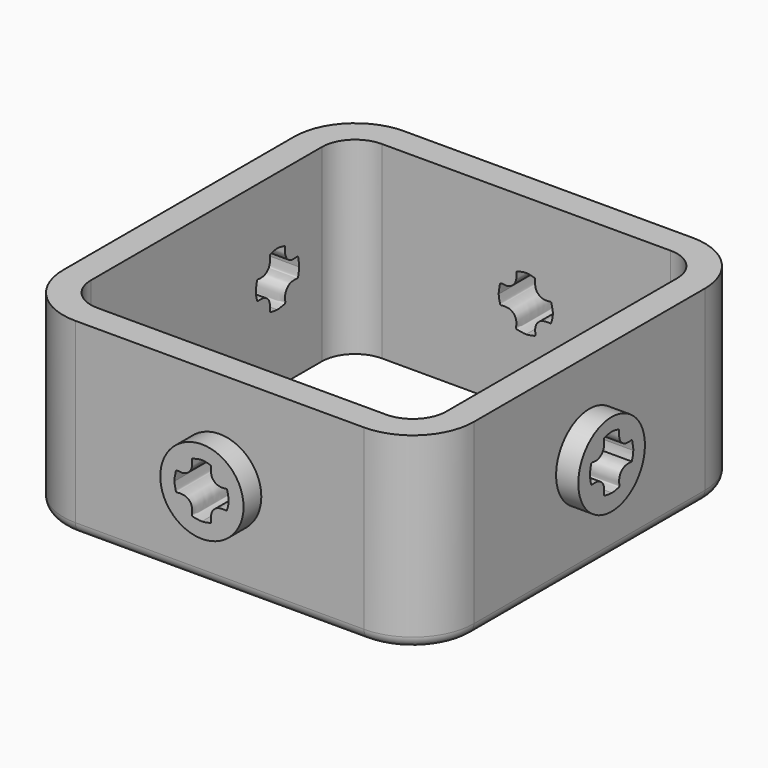
from build123d import *

# Parameters (mm, degrees)
F0_W      = 37
F0_H      = 37
F0_W_2    = 32
F0_H_2    = 32
F1_DEPTH  = 17
F2_R      = 3
F3_R      = 3.75
F4_DEPTH  = 2
F5_R      = 3.75
F6_DEPTH  = 2
F8_DEPTH  = 43.1
F9_R      = 5.5
F10_R     = 1
F12_DEPTH = 19.1
F13_R     = 3.75
F14_DEPTH = 2
F16_DEPTH = 25


# Not quite as in the source:
# - a pattern or mirror of a feature is missing from the dataset's text; its kind, count and spacing are read off the source's solid
# - a feature names something its author has since deleted; it is built from what else it names


with BuildPart() as f1:
    # F0 (on Top) → F1 (new body)
    with BuildSketch(Plane.XY):
        Rectangle(F0_W, F0_H)
        Rectangle(F0_W_2, F0_H_2, mode=Mode.SUBTRACT)
    extrude(amount=F1_DEPTH)

    # F2
    f2_edges = [f1.edges().sort_by_distance(p)[0] for p in [
        (-16, 16, 8.5),
        (16, 16, 8.5),
        (16, -16, 8.5),
        (-16, -16, 8.5),
    ]]
    fillet(f2_edges, radius=F2_R)

    # F3 (on face) → F4 (join)
    with BuildSketch(Plane(origin=(-18.5, 0, 0), x_dir=(0, -1, 0), z_dir=(-1, 0, 0))):
        with Locations((-8, 8.5)):
            Circle(F3_R)
        with BuildLine():
            ThreePointArc((11.75, 8.5), (8, 12.25), (4.25, 8.5))
            ThreePointArc((4.25, 8.5), (8, 4.75), (11.75, 8.5))
        make_face()
    extrude(amount=F4_DEPTH)

    # F5 (on face) → F6 (join)
    with BuildSketch(Plane.XZ.offset(18.5)):
        with Locations((0, 8.5)):
            Circle(F5_R)
    f6 = extrude(amount=F6_DEPTH)

    # F6_copies: F6 across plane
    add(f6.mirror(Plane.ZX))

    # F7 (on face) → F8 (cut)
    with BuildSketch(Plane.XZ.offset(20.5)):
        with BuildLine():
            add(Edge.make_bspline(
                [(-0.8818770875, 10.8338655923), (-0.5842589697, 10.9177265658), (-0.286617976, 11.0030384337), (0.0019111567, 11.0008564852)],
                knots=[0, 0, 0, 0, 0.5095712537, 0.5095712537, 0.5095712537, 0.5095712537], degree=3))
            add(Edge.make_bspline(
                [(-0.8818770875, 10.8338655923), (-0.8820201865, 10.7347613501), (-0.8822944124, 10.5448442864), (-0.8804438019, 10.2880725266), (-0.8966687632, 10.0993117062), (-1.068596367, 9.7410775604), (-1.2714231603, 9.5700618662), (-1.5485520687, 9.4347869785), (-1.8416222457, 9.3826988039), (-2.3755108047, 9.5150016948), (-2.3789289487, 9.1137847523), (-2.4627570935, 8.8526861228), (-2.4717232683, 8.6257526766), (-2.4694705272, 8.5165882094)],
                knots=[0, 0, 0, 0, 0.0273605905, 0.0524320947, 0.0745076412, 0.1056108167, 0.1318649214, 0.158948127, 0.1874687016, 0.220995097, 0.2482860623, 0.2755720453, 0.3045111481, 0.3045111481, 0.3045111481, 0.3045111481], degree=3))
            Line((-2.4694705272, 8.5165882094), (0.0019111567, 8.5165882094))
            Line((0.0019111567, 8.5165882094), (0.0019111567, 11.0008564852))
        make_face()
        with BuildLine():
            add(Edge.make_bspline(
                [(0.0019111567, 11.0008564852), (0.2796014301, 10.9987565035), (0.5488515745, 10.9156128039), (0.8181237458, 10.8338655923)],
                knots=[0.5095712537, 0.5095712537, 0.5095712537, 0.5095712537, 1, 1, 1, 1], degree=3))
            Line((0.0019111567, 11.0008564852), (0.0019111567, 8.5165882094))
            Line((0.0019111567, 8.5165882094), (2.4063107129, 8.5165882094))
            add(Edge.make_bspline(
                [(0.8181237458, 10.8338655923), (0.808573955, 10.6407431128), (0.7908958141, 10.2733540765), (0.9265490604, 9.8190069198), (1.2705426119, 9.5087658937), (1.613327195, 9.4034651855), (2.0228532874, 9.3941178531), (2.2768502469, 9.4678694205), (2.31476899, 9.1461468983), (2.4034798172, 8.8157557592), (2.4088888856, 8.6033558583), (2.4063107129, 8.5165882094)],
                knots=[0, 0, 0, 0, 0.1117445823, 0.2125923647, 0.3107430927, 0.4000660841, 0.4960442665, 0.5626441507, 0.6379036869, 0.7311412958, 0.7990460169, 0.7990460169, 0.7990460169, 0.7990460169], degree=3))
        make_face()
        with BuildLine():
            Line((2.4063107129, 8.5165882094), (0.0019111567, 8.5165882094))
            Line((0.0019111567, 8.5165882094), (0.0019111567, 6.1379039912))
            add(Edge.make_bspline(
                [(0.0019111567, 6.1379039912), (0.0880019036, 6.1384753422), (0.2673868808, 6.1419263908), (0.617437794, 6.2421060681), (0.8782709541, 6.2426630103), (0.8055886858, 6.6298380402), (0.8079793199, 6.8775378709), (0.9099548949, 7.2279927312), (1.051872297, 7.4164777555), (1.3219909517, 7.6492500111), (1.7482840093, 7.7308769803), (2.0714959652, 7.7189104891), (2.2392537458, 7.7126994812)],
                knots=[0.714256594, 0.714256594, 0.714256594, 0.714256594, 0.7402463844, 0.7710533559, 0.7932728015, 0.8216277676, 0.8482190477, 0.8777914221, 0.9023565188, 0.9315770045, 0.9644861842, 1, 1, 1, 1], degree=3))
            add(Edge.make_bspline(
                [(2.4063107129, 8.5165882094), (2.4055950736, 8.4925035772), (2.3996248213, 8.3617285128), (2.3722923332, 8.1200925705), (2.2851858421, 7.8550741153), (2.2392537458, 7.7126994812)],
                knots=[0.7990460169, 0.7990460169, 0.7990460169, 0.7990460169, 0.8178947498, 0.9022950941, 1, 1, 1, 1], degree=3))
        make_face()
        with BuildLine():
            Line((0.0019111567, 8.5165882094), (-2.4694705272, 8.5165882094))
            add(Edge.make_bspline(
                [(-2.4694705272, 8.5165882094), (-2.4673672521, 8.4146666453), (-2.4513922887, 8.2265508139), (-2.378101265, 7.9832109794), (-2.3433019396, 7.6529651458), (-2.0959578633, 7.7306809949), (-1.79570178, 7.7162168111), (-1.543783127, 7.6842300062), (-1.3539542471, 7.6082528592), (-1.1255377786, 7.4279201775), (-1.0230772684, 7.2863305188), (-0.9248223588, 7.1065020744), (-0.8786532076, 6.8480078897), (-0.865803798, 6.6232555694), (-0.9578786763, 6.2310932538), (-0.605902395, 6.223767445), (-0.282541062, 6.1383204524), (-0.0861655165, 6.1373194605), (0.0019111567, 6.1379039912)],
                knots=[0.3045111481, 0.3045111481, 0.3045111481, 0.3045111481, 0.3315301836, 0.3578655515, 0.3837385363, 0.4059679792, 0.434252013, 0.4594532962, 0.4822711791, 0.5090972104, 0.530231005, 0.5527300135, 0.5781274322, 0.6031996615, 0.6315546276, 0.6576667534, 0.6876672756, 0.714256594, 0.714256594, 0.714256594, 0.714256594], degree=3))
            Line((0.0019111567, 6.1379039912), (0.0019111567, 8.5165882094))
        make_face()
    extrude(amount=-F8_DEPTH, mode=Mode.SUBTRACT)

    # F9
    f9_edges = [f1.edges().sort_by_distance(p)[0] for p in [
        (-18.5, -18.5, 8.5),
        (18.5, -18.5, 8.5),
        (18.5, 18.5, 8.5),
        (-18.5, 18.5, 8.5),
    ]]
    fillet(f9_edges, radius=F9_R)

    # F10
    f10_edges = [f1.edges().sort_by_distance(p)[0] for p in [
        (18.5, 0, 0),
        (-16.889087, -16.889087, 0),
        (0, -18.5, 0),
        (16.889087, -16.889087, 0),
        (-18.5, 0, 0),
        (-16.889087, 16.889087, 0),
        (0, 18.5, 0),
        (16.889087, 16.889087, 0),
    ]]
    fillet(f10_edges, radius=F10_R)

    # F11 (on face) → F12 (cut)
    with BuildSketch(Plane(origin=(-20.5, 0, 0), x_dir=(0, -1, 0), z_dir=(-1, 0, 0))):
        with BuildLine():
            add(Edge.make_bspline(
                [(-8.8643170893, 10.8358810569), (-8.5666989715, 10.9197420305), (-8.2690579778, 11.0050538983), (-7.9805288451, 11.0028719498)],
                knots=[0, 0, 0, 0, 0.5095712537, 0.5095712537, 0.5095712537, 0.5095712537], degree=3))
            add(Edge.make_bspline(
                [(-8.8643170893, 10.8358810569), (-8.8644601883, 10.7367768147), (-8.8647344142, 10.546859751), (-8.8628838037, 10.2900879912), (-8.879108765, 10.1013271709), (-9.0510363688, 9.743093025), (-9.2538631621, 9.5720773308), (-9.5309920705, 9.4368024432), (-9.8240622475, 9.3847142685), (-10.3579508065, 9.5170171595), (-10.3613689505, 9.1158002169), (-10.4451970953, 8.8547015875), (-10.4541632701, 8.6277681413), (-10.451910529, 8.5186036741)],
                knots=[0, 0, 0, 0, 0.0273605905, 0.0524320947, 0.0745076412, 0.1056108167, 0.1318649214, 0.158948127, 0.1874687016, 0.220995097, 0.2482860623, 0.2755720453, 0.3045111481, 0.3045111481, 0.3045111481, 0.3045111481], degree=3))
            Line((-10.451910529, 8.5186036741), (-7.9805288451, 8.5186036741))
            Line((-7.9805288451, 8.5186036741), (-7.9805288451, 11.0028719498))
        make_face()
        with BuildLine():
            add(Edge.make_bspline(
                [(-7.9805288451, 11.0028719498), (-7.7028385717, 11.0007719681), (-7.4335884273, 10.9176282686), (-7.164316256, 10.8358810569)],
                knots=[0.5095712537, 0.5095712537, 0.5095712537, 0.5095712537, 1, 1, 1, 1], degree=3))
            Line((-7.9805288451, 11.0028719498), (-7.9805288451, 8.5186036741))
            Line((-7.9805288451, 8.5186036741), (-5.5761292889, 8.5186036741))
            add(Edge.make_bspline(
                [(-7.164316256, 10.8358810569), (-7.1738660468, 10.6427585775), (-7.1915441877, 10.2753695412), (-7.0558909414, 9.8210223844), (-6.7118973899, 9.5107813584), (-6.3691128068, 9.4054806501), (-5.9595867144, 9.3961333178), (-5.7055897549, 9.4698848851), (-5.6676710118, 9.148162363), (-5.5789601846, 8.8177712239), (-5.5735511162, 8.6053713229), (-5.5761292889, 8.5186036741)],
                knots=[0, 0, 0, 0, 0.1117445823, 0.2125923647, 0.3107430927, 0.4000660841, 0.4960442665, 0.5626441507, 0.6379036869, 0.7311412958, 0.7990460169, 0.7990460169, 0.7990460169, 0.7990460169], degree=3))
        make_face()
        with BuildLine():
            Line((-5.5761292889, 8.5186036741), (-7.9805288451, 8.5186036741))
            Line((-7.9805288451, 8.5186036741), (-7.9805288451, 6.1399194559))
            add(Edge.make_bspline(
                [(-7.9805288451, 6.1399194559), (-7.8944380982, 6.1404908068), (-7.715053121, 6.1439418554), (-7.3650022078, 6.2441215327), (-7.1041690477, 6.2446784749), (-7.176851316, 6.6318535049), (-7.1744606819, 6.8795533355), (-7.0724851069, 7.2300081958), (-6.9305677048, 7.4184932202), (-6.6604490501, 7.6512654757), (-6.2341559925, 7.732892445), (-5.9109440366, 7.7209259537), (-5.743186256, 7.7147149458)],
                knots=[0.714256594, 0.714256594, 0.714256594, 0.714256594, 0.7402463844, 0.7710533559, 0.7932728015, 0.8216277676, 0.8482190477, 0.8777914221, 0.9023565188, 0.9315770045, 0.9644861842, 1, 1, 1, 1], degree=3))
            add(Edge.make_bspline(
                [(-5.5761292889, 8.5186036741), (-5.5768449282, 8.4945190419), (-5.5828151805, 8.3637439775), (-5.6101476686, 8.1221080351), (-5.6972541597, 7.85708958), (-5.743186256, 7.7147149458)],
                knots=[0.7990460169, 0.7990460169, 0.7990460169, 0.7990460169, 0.8178947498, 0.9022950941, 1, 1, 1, 1], degree=3))
        make_face()
        with BuildLine():
            Line((-7.9805288451, 8.5186036741), (-10.451910529, 8.5186036741))
            add(Edge.make_bspline(
                [(-10.451910529, 8.5186036741), (-10.4498072539, 8.41668211), (-10.4338322905, 8.2285662786), (-10.3605412668, 7.985226444), (-10.3257419414, 7.6549806105), (-10.0783978651, 7.7326964595), (-9.7781417818, 7.7182322757), (-9.5262231288, 7.6862454709), (-9.3363942489, 7.6102683238), (-9.1079777804, 7.4299356422), (-9.0055172702, 7.2883459835), (-8.9072623606, 7.108517539), (-8.8610932094, 6.8500233544), (-8.8482437998, 6.625271034), (-8.9403186781, 6.2331087185), (-8.5883423968, 6.2257829096), (-8.2649810638, 6.140335917), (-8.0686055183, 6.1393349251), (-7.9805288451, 6.1399194559)],
                knots=[0.3045111481, 0.3045111481, 0.3045111481, 0.3045111481, 0.3315301836, 0.3578655515, 0.3837385363, 0.4059679792, 0.434252013, 0.4594532962, 0.4822711791, 0.5090972104, 0.530231005, 0.5527300135, 0.5781274322, 0.6031996615, 0.6315546276, 0.6576667534, 0.6876672756, 0.714256594, 0.714256594, 0.714256594, 0.714256594], degree=3))
            Line((-7.9805288451, 6.1399194559), (-7.9805288451, 8.5186036741))
        make_face()
        with BuildLine():
            add(Edge.make_bspline(
                [(7.1871276014, 10.8358810569), (7.4847457192, 10.9197420305), (7.7823867129, 11.0050538983), (8.0709158455, 11.0028719498)],
                knots=[0, 0, 0, 0, 0.5095712537, 0.5095712537, 0.5095712537, 0.5095712537], degree=3))
            add(Edge.make_bspline(
                [(7.1871276014, 10.8358810569), (7.1869845023, 10.7367768147), (7.1867102765, 10.546859751), (7.188560887, 10.2900879912), (7.1723359257, 10.1013271709), (7.0004083219, 9.743093025), (6.7975815286, 9.5720773308), (6.5204526202, 9.4368024432), (6.2273824431, 9.3847142685), (5.6934938842, 9.5170171595), (5.6900757401, 9.1158002169), (5.6062475953, 8.8547015875), (5.5972814206, 8.6277681413), (5.5995341617, 8.5186036741)],
                knots=[0, 0, 0, 0, 0.0273605905, 0.0524320947, 0.0745076412, 0.1056108167, 0.1318649214, 0.158948127, 0.1874687016, 0.220995097, 0.2482860623, 0.2755720453, 0.3045111481, 0.3045111481, 0.3045111481, 0.3045111481], degree=3))
            Line((5.5995341617, 8.5186036741), (8.0709158455, 8.5186036741))
            Line((8.0709158455, 8.5186036741), (8.0709158455, 11.0028719498))
        make_face()
        with BuildLine():
            add(Edge.make_bspline(
                [(8.0709158455, 11.0028719498), (8.348606119, 11.0007719681), (8.6178562634, 10.9176282686), (8.8871284347, 10.8358810569)],
                knots=[0.5095712537, 0.5095712537, 0.5095712537, 0.5095712537, 1, 1, 1, 1], degree=3))
            Line((8.0709158455, 11.0028719498), (8.0709158455, 8.5186036741))
            Line((8.0709158455, 8.5186036741), (10.4753154018, 8.5186036741))
            add(Edge.make_bspline(
                [(8.8871284347, 10.8358810569), (8.8775786439, 10.6427585775), (8.859900503, 10.2753695412), (8.9955537493, 9.8210223844), (9.3395473008, 9.5107813584), (9.6823318839, 9.4054806501), (10.0918579763, 9.3961333178), (10.3458549357, 9.4698848851), (10.3837736789, 9.148162363), (10.4724845061, 8.8177712239), (10.4778935745, 8.6053713229), (10.4753154018, 8.5186036741)],
                knots=[0, 0, 0, 0, 0.1117445823, 0.2125923647, 0.3107430927, 0.4000660841, 0.4960442665, 0.5626441507, 0.6379036869, 0.7311412958, 0.7990460169, 0.7990460169, 0.7990460169, 0.7990460169], degree=3))
        make_face()
        with BuildLine():
            Line((10.4753154018, 8.5186036741), (8.0709158455, 8.5186036741))
            Line((8.0709158455, 8.5186036741), (8.0709158455, 6.1399194559))
            add(Edge.make_bspline(
                [(8.0709158455, 6.1399194559), (8.1570065925, 6.1404908068), (8.3363915697, 6.1439418554), (8.6864424829, 6.2441215327), (8.947275643, 6.2446784749), (8.8745933747, 6.6318535049), (8.8769840088, 6.8795533355), (8.9789595838, 7.2300081958), (9.1208769859, 7.4184932202), (9.3909956405, 7.6512654757), (9.8172886982, 7.732892445), (10.140500654, 7.7209259537), (10.3082584347, 7.7147149458)],
                knots=[0.714256594, 0.714256594, 0.714256594, 0.714256594, 0.7402463844, 0.7710533559, 0.7932728015, 0.8216277676, 0.8482190477, 0.8777914221, 0.9023565188, 0.9315770045, 0.9644861842, 1, 1, 1, 1], degree=3))
            add(Edge.make_bspline(
                [(10.4753154018, 8.5186036741), (10.4745997624, 8.4945190419), (10.4686295102, 8.3637439775), (10.4412970221, 8.1221080351), (10.354190531, 7.85708958), (10.3082584347, 7.7147149458)],
                knots=[0.7990460169, 0.7990460169, 0.7990460169, 0.7990460169, 0.8178947498, 0.9022950941, 1, 1, 1, 1], degree=3))
        make_face()
        with BuildLine():
            Line((8.0709158455, 8.5186036741), (5.5995341617, 8.5186036741))
            add(Edge.make_bspline(
                [(5.5995341617, 8.5186036741), (5.6016374367, 8.41668211), (5.6176124001, 8.2285662786), (5.6909034238, 7.985226444), (5.7257027493, 7.6549806105), (5.9730468256, 7.7326964595), (6.2733029089, 7.7182322757), (6.5252215619, 7.6862454709), (6.7150504418, 7.6102683238), (6.9434669103, 7.4299356422), (7.0459274204, 7.2883459835), (7.1441823301, 7.108517539), (7.1903514813, 6.8500233544), (7.2032008909, 6.625271034), (7.1111260125, 6.2331087185), (7.4631022939, 6.2257829096), (7.7864636269, 6.140335917), (7.9828391724, 6.1393349251), (8.0709158455, 6.1399194559)],
                knots=[0.3045111481, 0.3045111481, 0.3045111481, 0.3045111481, 0.3315301836, 0.3578655515, 0.3837385363, 0.4059679792, 0.434252013, 0.4594532962, 0.4822711791, 0.5090972104, 0.530231005, 0.5527300135, 0.5781274322, 0.6031996615, 0.6315546276, 0.6576667534, 0.6876672756, 0.714256594, 0.714256594, 0.714256594, 0.714256594], degree=3))
            Line((8.0709158455, 6.1399194559), (8.0709158455, 8.5186036741))
        make_face()
    extrude(amount=-F12_DEPTH, mode=Mode.SUBTRACT)

    # F13 (on face) → F14 (join)
    with BuildSketch(Plane.YZ.offset(18.5)):
        with Locations((0, 9)):
            Circle(F13_R)
    extrude(amount=F14_DEPTH)

    # F15 (on face) → F16 (cut)
    with BuildSketch(Plane.YZ.offset(20.5)):
        with BuildLine():
            add(Edge.make_bspline(
                [(-0.8486843435, 11.4162178162), (-0.5510662257, 11.5000787897), (-0.253425232, 11.5853906576), (0.0351039007, 11.583208709)],
                knots=[0, 0, 0, 0, 0.5095712537, 0.5095712537, 0.5095712537, 0.5095712537], degree=3))
            add(Edge.make_bspline(
                [(-0.8486843435, 11.4162178162), (-0.8488274425, 11.3171135739), (-0.8491016684, 11.1271965102), (-0.8472510579, 10.8704247505), (-0.8634760192, 10.6816639301), (-1.035403623, 10.3234297843), (-1.2382304163, 10.15241409), (-1.5153593247, 10.0171392024), (-1.8084295017, 9.9650510278), (-2.3423180606, 10.0973539187), (-2.3457362047, 9.6961369761), (-2.4295643495, 9.4350383467), (-2.4385305242, 9.2081049005), (-2.4362777831, 9.0989404333)],
                knots=[0, 0, 0, 0, 0.0273605905, 0.0524320947, 0.0745076412, 0.1056108167, 0.1318649214, 0.158948127, 0.1874687016, 0.220995097, 0.2482860623, 0.2755720453, 0.3045111481, 0.3045111481, 0.3045111481, 0.3045111481], degree=3))
            Line((-2.4362777831, 9.0989404333), (0.0351039007, 9.0989404333))
            Line((0.0351039007, 9.0989404333), (0.0351039007, 11.583208709))
        make_face()
        with BuildLine():
            add(Edge.make_bspline(
                [(0.0351039007, 11.583208709), (0.3127941741, 11.5811087274), (0.5820443186, 11.4979650278), (0.8513164898, 11.4162178162)],
                knots=[0.5095712537, 0.5095712537, 0.5095712537, 0.5095712537, 1, 1, 1, 1], degree=3))
            Line((0.0351039007, 11.583208709), (0.0351039007, 9.0989404333))
            Line((0.0351039007, 9.0989404333), (2.4395034569, 9.0989404333))
            add(Edge.make_bspline(
                [(0.8513164898, 11.4162178162), (0.841766699, 11.2230953367), (0.8240885581, 10.8557063004), (0.9597418044, 10.4013591437), (1.3037353559, 10.0911181176), (1.646519939, 9.9858174093), (2.0560460314, 9.976470077), (2.3100429909, 10.0502216443), (2.347961734, 9.7284991222), (2.4366725612, 9.3981079831), (2.4420816296, 9.1857080821), (2.4395034569, 9.0989404333)],
                knots=[0, 0, 0, 0, 0.1117445823, 0.2125923647, 0.3107430927, 0.4000660841, 0.4960442665, 0.5626441507, 0.6379036869, 0.7311412958, 0.7990460169, 0.7990460169, 0.7990460169, 0.7990460169], degree=3))
        make_face()
        with BuildLine():
            Line((2.4395034569, 9.0989404333), (0.0351039007, 9.0989404333))
            Line((0.0351039007, 9.0989404333), (0.0351039007, 6.7202562151))
            add(Edge.make_bspline(
                [(0.0351039007, 6.7202562151), (0.1211946476, 6.720827566), (0.3005796248, 6.7242786147), (0.6506305381, 6.8244582919), (0.9114636981, 6.8250152341), (0.8387814298, 7.2121902641), (0.8411720639, 7.4598900948), (0.9431476389, 7.810344955), (1.085065041, 7.9988299794), (1.3551836957, 8.2316022349), (1.7814767533, 8.3132292042), (2.1046887092, 8.301262713), (2.2724464898, 8.295051705)],
                knots=[0.714256594, 0.714256594, 0.714256594, 0.714256594, 0.7402463844, 0.7710533559, 0.7932728015, 0.8216277676, 0.8482190477, 0.8777914221, 0.9023565188, 0.9315770045, 0.9644861842, 1, 1, 1, 1], degree=3))
            add(Edge.make_bspline(
                [(2.4395034569, 9.0989404333), (2.4387878176, 9.0748558011), (2.4328175653, 8.9440807367), (2.4054850772, 8.7024447943), (2.3183785861, 8.4374263392), (2.2724464898, 8.295051705)],
                knots=[0.7990460169, 0.7990460169, 0.7990460169, 0.7990460169, 0.8178947498, 0.9022950941, 1, 1, 1, 1], degree=3))
        make_face()
        with BuildLine():
            Line((0.0351039007, 9.0989404333), (-2.4362777831, 9.0989404333))
            add(Edge.make_bspline(
                [(-2.4362777831, 9.0989404333), (-2.4341745081, 8.9970188692), (-2.4181995447, 8.8089030378), (-2.344908521, 8.5655632032), (-2.3101091956, 8.2353173697), (-2.0627651192, 8.3130332188), (-1.7625090359, 8.2985690349), (-1.510590383, 8.2665822301), (-1.3207615031, 8.1906050831), (-1.0923450346, 8.0102724014), (-0.9898845244, 7.8686827427), (-0.8916296148, 7.6888542982), (-0.8454604636, 7.4303601136), (-0.8326110539, 7.2056077932), (-0.9246859323, 6.8134454777), (-0.572709651, 6.8061196688), (-0.249348318, 6.7206726762), (-0.0529727725, 6.7196716844), (0.0351039007, 6.7202562151)],
                knots=[0.3045111481, 0.3045111481, 0.3045111481, 0.3045111481, 0.3315301836, 0.3578655515, 0.3837385363, 0.4059679792, 0.434252013, 0.4594532962, 0.4822711791, 0.5090972104, 0.530231005, 0.5527300135, 0.5781274322, 0.6031996615, 0.6315546276, 0.6576667534, 0.6876672756, 0.714256594, 0.714256594, 0.714256594, 0.714256594], degree=3))
            Line((0.0351039007, 6.7202562151), (0.0351039007, 9.0989404333))
        make_face()
    extrude(amount=-F16_DEPTH, mode=Mode.SUBTRACT)


solid = f1.part
